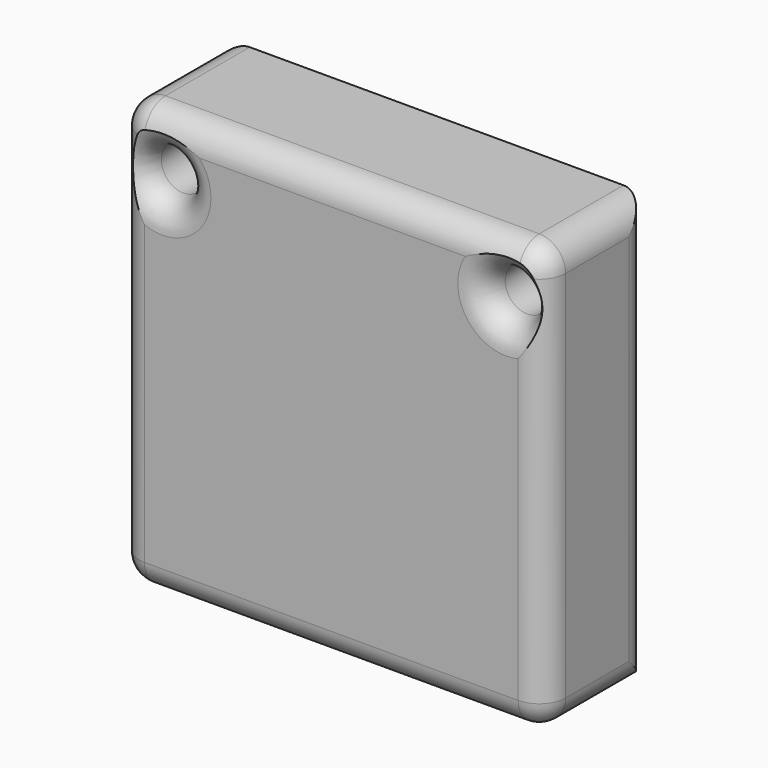
from build123d import *

# Parameters (mm, degrees)
F0_W         = 82.2881497443
F0_H         = 82.288146019
F0_R         = 4.2853217598
F1_DEPTH     = 25.4
F2_T1_DEPTH  = 33.02
F2_T3_DEPTH  = 107.688146019
F2_T5_DEPTH  = 72.128146019
F2_T7_DEPTH  = 72.1281497443
F2_S11_W     = 5.08
F2_S11_H     = 5.08
F2_T12_DEPTH = 5.08
F2_S17_W     = 5.08
F2_S17_H     = 5.08
F2_T18_DEPTH = 5.08
F2_S23_W     = 5.08
F2_S23_H     = 5.08
F2_T24_DEPTH = 5.08
F2_S29_W     = 5.08
F2_S29_H     = 5.08
F2_T30_DEPTH = 5.08


# Not quite as in the source:
# - a fillet or chamfer that OpenCascade refuses, or shapes differently, is made with other operations: its cross-section is extruded or revolved along the edge and cut away or added
# - a feature of the source that left no trace in its solid (it failed there, or was rolled back) is left out


with BuildPart() as f1:
    # F0 (on Front) → F1 (new body)
    with BuildSketch(Plane.XZ):
        with Locations((2.3490097374, -1.9460879266)):
            Rectangle(F0_W, F0_H)
        with Locations((-30.2557293326, 28.0709732324)):
            Circle(F0_R, mode=Mode.SUBTRACT)
        with Locations((36.1182056367, 29.1060488671)):
            Circle(F0_R, mode=Mode.SUBTRACT)
    extrude(amount=F1_DEPTH)

    # F2: fillet of radius 5.08 on 12 edges, made by hand

    # F2_s2 → F2_t1 (cut)
    with BuildSketch(Plane.XZ.offset(-12.7)):
        with BuildLine():
            ThreePointArc((38.4130846095, -43.0901609361), (42.0051870579, -41.6022633845), (43.4930846095, -38.0101609361))
            Line((43.4930846095, -38.0101609361), (43.4930846095, -43.0901609361))
            Line((43.4930846095, -43.0901609361), (38.4130846095, -43.0901609361))
        make_face()
        with BuildLine():
            ThreePointArc((38.4130846095, 39.1979850829), (42.0051870579, 37.7100875313), (43.4930846095, 34.1179850829))
            Line((43.4930846095, 34.1179850829), (43.4930846095, 39.1979850829))
            Line((43.4930846095, 39.1979850829), (38.4130846095, 39.1979850829))
        make_face()
        with BuildLine():
            ThreePointArc((-33.7150651348, 39.1979850829), (-37.3071675832, 37.7100875313), (-38.7950651348, 34.1179850829))
            Line((-38.7950651348, 34.1179850829), (-38.7950651348, 39.1979850829))
            Line((-38.7950651348, 39.1979850829), (-33.7150651348, 39.1979850829))
        make_face()
        with BuildLine():
            ThreePointArc((-38.7950651348, -38.0101609361), (-37.3071675832, -41.6022633845), (-33.7150651348, -43.0901609361))
            Line((-33.7150651348, -43.0901609361), (-38.7950651348, -43.0901609361))
            Line((-38.7950651348, -43.0901609361), (-38.7950651348, -38.0101609361))
        make_face()
    extrude(amount=F2_T1_DEPTH, mode=Mode.SUBTRACT)

    # F2_s4 → F2_t3 (cut)
    with BuildSketch(Plane.XY.offset(-55.7901609361)):
        with BuildLine():
            ThreePointArc((43.4930846095, -5.08), (42.0051870579, -1.4878975516), (38.4130846095, 0))
            Line((38.4130846095, 0), (43.4930846095, 0))
            Line((43.4930846095, 0), (43.4930846095, -5.08))
        make_face()
        with BuildLine():
            ThreePointArc((-38.7950651348, -5.08), (-37.3071675832, -1.4878975516), (-33.7150651348, 0))
            Line((-33.7150651348, 0), (-38.7950651348, 0))
            Line((-38.7950651348, 0), (-38.7950651348, -5.08))
        make_face()
    extrude(amount=F2_T3_DEPTH, mode=Mode.SUBTRACT)

    # F2_s6 → F2_t5 (cut)
    with BuildSketch(Plane.XY.offset(-38.0101609361)):
        with BuildLine():
            ThreePointArc((43.4930846095, -20.32), (42.0051870579, -23.9121024484), (38.4130846095, -25.4))
            Line((38.4130846095, -25.4), (43.4930846095, -25.4))
            Line((43.4930846095, -25.4), (43.4930846095, -20.32))
        make_face()
        with BuildLine():
            ThreePointArc((-38.7950651348, -20.32), (-37.3071675832, -23.9121024484), (-33.7150651348, -25.4))
            Line((-33.7150651348, -25.4), (-38.7950651348, -25.4))
            Line((-38.7950651348, -25.4), (-38.7950651348, -20.32))
        make_face()
    extrude(amount=F2_T5_DEPTH, mode=Mode.SUBTRACT)

    # F2_s8 → F2_t7 (cut)
    with BuildSketch(Plane.YZ.offset(-33.7150651348)):
        with BuildLine():
            ThreePointArc((-20.32, 39.1979850829), (-23.9121024484, 37.7100875313), (-25.4, 34.1179850829))
            Line((-25.4, 34.1179850829), (-25.4, 39.1979850829))
            Line((-25.4, 39.1979850829), (-20.32, 39.1979850829))
        make_face()
        with BuildLine():
            ThreePointArc((-20.32, -43.0901609361), (-23.9121024484, -41.6022633845), (-25.4, -38.0101609361))
            Line((-25.4, -38.0101609361), (-25.4, -43.0901609361))
            Line((-25.4, -43.0901609361), (-20.32, -43.0901609361))
        make_face()
    extrude(amount=F2_T7_DEPTH, mode=Mode.SUBTRACT)


with BuildPart() as f2_tool10:
    # F2_s11 → F2_t12 (new body)
    with BuildSketch(Plane.XY.offset(-38.0101609361)):
        with Locations((40.9530846095, -22.86)):
            Rectangle(F2_S11_W, F2_S11_H)
    extrude(amount=-F2_T12_DEPTH)

    # F2_s13 → F2_t14 (revolve, cut)
    with BuildSketch(Plane(origin=(38.4130846095, -20.32, -38.0101609361), x_dir=(-0.7071067812, 0.7071067812, 0), z_dir=(-0.7071067812, -0.7071067812, 0))):
        with BuildLine():
            ThreePointArc((0, -5.08), (5.08, 0), (0, 5.08))
            Line((0, 5.08), (0, -5.08))
        make_face()
    revolve(axis=Axis((38.4130846095, -20.32, -38.0101609361), (0, 0, -1)), mode=Mode.SUBTRACT)


with BuildPart() as f1_1:
    add(f1.part)

    # F2_t9: cut F2_tool10
    add(f2_tool10.part, mode=Mode.SUBTRACT)


with BuildPart() as f2_tool16:
    # F2_s17 → F2_t18 (new body)
    with BuildSketch(Plane.XY.offset(34.1179850829)):
        with Locations((40.9530846095, -22.86)):
            Rectangle(F2_S17_W, F2_S17_H)
    extrude(amount=F2_T18_DEPTH)

    # F2_s19 → F2_t20 (revolve, cut)
    with BuildSketch(Plane(origin=(38.4130846095, -20.32, 34.1179850829), x_dir=(-0.7071067812, 0.7071067812, 0), z_dir=(0.7071067812, 0.7071067812, 0))):
        with BuildLine():
            ThreePointArc((0, -5.08), (5.08, 0), (0, 5.08))
            Line((0, 5.08), (0, -5.08))
        make_face()
    revolve(axis=Axis((38.4130846095, -20.32, 34.1179850829), (0, 0, 1)), mode=Mode.SUBTRACT)


with BuildPart() as f1_2:
    add(f1_1.part)

    # F2_t15: cut F2_tool16
    add(f2_tool16.part, mode=Mode.SUBTRACT)


with BuildPart() as f2_tool22:
    # F2_s23 → F2_t24 (new body)
    with BuildSketch(Plane.XY.offset(34.1179850829)):
        with Locations((-36.2550651348, -22.86)):
            Rectangle(F2_S23_W, F2_S23_H)
    extrude(amount=F2_T24_DEPTH)

    # F2_s25 → F2_t26 (revolve, cut)
    with BuildSketch(Plane(origin=(-33.7150651348, -20.32, 34.1179850829), x_dir=(0.7071067812, 0.7071067812, 0), z_dir=(0.7071067812, -0.7071067812, 0))):
        with BuildLine():
            ThreePointArc((0, -5.08), (5.08, 0), (0, 5.08))
            Line((0, 5.08), (0, -5.08))
        make_face()
    revolve(axis=Axis((-33.7150651348, -20.32, 34.1179850829), (0, 0, 1)), mode=Mode.SUBTRACT)


with BuildPart() as f1_3:
    add(f1_2.part)

    # F2_t21: cut F2_tool22
    add(f2_tool22.part, mode=Mode.SUBTRACT)


with BuildPart() as f2_tool28:
    # F2_s29 → F2_t30 (new body)
    with BuildSketch(Plane.YZ.offset(-33.7150651348)):
        with Locations((-22.86, -40.5501609361)):
            Rectangle(F2_S29_W, F2_S29_H)
    extrude(amount=-F2_T30_DEPTH)

    # F2_s31 → F2_t32 (revolve, cut)
    with BuildSketch(Plane(origin=(-33.7150651348, -20.32, -38.0101609361), x_dir=(0, 0.7071067812, 0.7071067812), z_dir=(0, -0.7071067812, 0.7071067812))):
        with BuildLine():
            ThreePointArc((0, -5.08), (5.08, 0), (0, 5.08))
            Line((0, 5.08), (0, -5.08))
        make_face()
    revolve(axis=Axis((-33.7150651348, -20.32, -38.0101609361), (-1, 0, 0)), mode=Mode.SUBTRACT)


with BuildPart() as f1_4:
    add(f1_3.part)

    # F2_t27: cut F2_tool28
    add(f2_tool28.part, mode=Mode.SUBTRACT)

    # F2_s33 → F2_t34 (revolve, cut)
    with BuildSketch(Plane.XY.offset(28.0709732324)):
        with BuildLine():
            ThreePointArc((-25.9704075728, -20.32), (-24.4825100212, -23.9121024484), (-20.8904075728, -25.4))
            Line((-20.8904075728, -25.4), (-25.9704075728, -25.4))
            Line((-25.9704075728, -25.4), (-25.9704075728, -20.32))
        make_face()
    revolve(axis=Axis((-30.2557293326, -25.4, 28.0709732324), (0, -1, 0)), mode=Mode.SUBTRACT)

    # F2_s35 → F2_t36 (revolve, cut)
    with BuildSketch(Plane.XY.offset(29.1060488671)):
        with BuildLine():
            ThreePointArc((40.4035273965, -20.32), (41.8914249481, -23.9121024484), (45.4835273965, -25.4))
            Line((45.4835273965, -25.4), (40.4035273965, -25.4))
            Line((40.4035273965, -25.4), (40.4035273965, -20.32))
        make_face()
    revolve(axis=Axis((36.1182056367, -25.4, 29.1060488671), (0, -1, 0)), mode=Mode.SUBTRACT)


solid = f1_4.part
